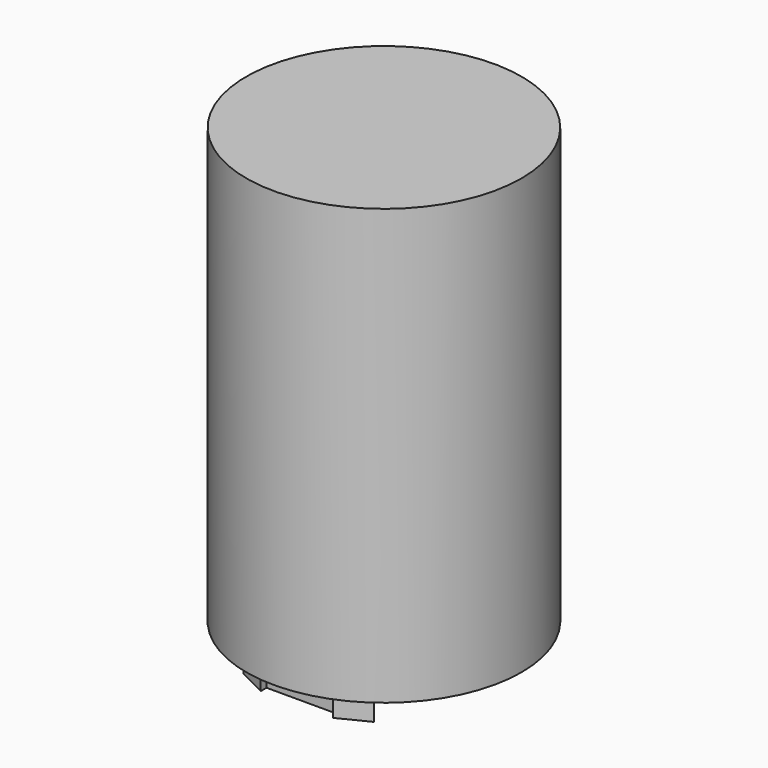
from build123d import *

# Parameters (mm, degrees)
F1_DEPTH = 2
F0_R     = 9.5
F2_DEPTH = 30


with BuildPart() as f1:
    # F0 (on Top) → F1 (new body)
    with BuildSketch(Plane.XY):
        with BuildLine():
            Line((-2.5, -4.5), (-1.5, -4.5))
            Line((-1.5, -4.5), (-1.5, 8))
            ThreePointArc((-1.5, 8), (-1.8805656371, 8.4555551787), (-2.3965696716, 8.1621262073))
            Line((-2.3965696716, 8.1621262073), (-7.1307446703, -4.5))
            Line((-7.1307446703, -4.5), (-6.1307446703, -4.5))
            Line((-6.1307446703, -4.5), (-5.1960329715, -2))
            Line((-5.1960329715, -2), (-2.5, -2))
            Line((-2.5, -2), (-2.5, -4.5))
        make_face()
        Polygon((-2.5, -1), (-4.8221482921, -1), (-2.5, 5.210867734), align=None, mode=Mode.SUBTRACT)
    extrude(amount=-F1_DEPTH)


with BuildPart() as f1b:
    # F0 (on Top) → F1, piece 2 (new body)
    with BuildSketch(Plane.XY):
        with BuildLine():
            Line((1.5, 8.4555551787), (1.5, -4.5))
            ThreePointArc((1.5, -4.5), (5.317050605, -1.9109756291), (7, 2.3832767911))
            ThreePointArc((7, 2.3832767911), (5.154069353, 6.2382818411), (1.5, 8.4555551787))
        make_face()
        Polygon((2.5, -3.0675162561), (2.5, 7.2462004609), (6.0021702136, 2.449122956), align=None, mode=Mode.SUBTRACT)
    extrude(amount=-F1_DEPTH)


with BuildPart() as f1c:
    # F0 (on Top) → F1, piece 3 (new body)
    with BuildSketch(Plane.XY):
        Polygon((2.5, -6), (-2.5, -6), (-2.5, -5.5), (-4.5, -6.5), (-2.5, -7.5), (-2.5, -7), (2.5, -7), (2.5, -7.5), (4.5, -6.5), (2.5, -5.5), align=None)
    extrude(amount=-F1_DEPTH)


with BuildPart() as f2:
    # F0 (on Top) → F2 (new body)
    with BuildSketch(Plane.XY):
        Circle(F0_R)
        Polygon((-2.5, -5.5), (-2.5, -6), (2.5, -6), (2.5, -5.5), (4.5, -6.5), (2.5, -7.5), (2.5, -7), (-2.5, -7), (-2.5, -7.5), (-4.5, -6.5), align=None, mode=Mode.SUBTRACT)
        with BuildLine():
            Line((-1.5, 8), (-1.5, -4.5))
            Line((-1.5, -4.5), (-2.5, -4.5))
            Line((-2.5, -4.5), (-2.5, -2))
            Line((-2.5, -2), (-5.1960329715, -2))
            Line((-5.1960329715, -2), (-6.1307446703, -4.5))
            Line((-6.1307446703, -4.5), (-7.1307446703, -4.5))
            Line((-7.1307446703, -4.5), (-2.3965696716, 8.1621262073))
            ThreePointArc((-2.3965696716, 8.1621262073), (-1.8805656371, 8.4555551787), (-1.5, 8))
        make_face(mode=Mode.SUBTRACT)
        with BuildLine():
            ThreePointArc((7, 2.3832767911), (5.317050605, -1.9109756291), (1.5, -4.5))
            Line((1.5, -4.5), (1.5, 8.4555551787))
            ThreePointArc((1.5, 8.4555551787), (5.154069353, 6.2382818411), (7, 2.3832767911))
        make_face(mode=Mode.SUBTRACT)
        with BuildLine():
            Line((1.5, 8.4555551787), (1.5, -4.5))
            ThreePointArc((1.5, -4.5), (5.317050605, -1.9109756291), (7, 2.3832767911))
            ThreePointArc((7, 2.3832767911), (5.154069353, 6.2382818411), (1.5, 8.4555551787))
        make_face()
        Polygon((2.5, -3.0675162561), (2.5, 7.2462004609), (6.0021702136, 2.449122956), align=None, mode=Mode.SUBTRACT)
        with BuildLine():
            Line((-2.5, -4.5), (-1.5, -4.5))
            Line((-1.5, -4.5), (-1.5, 8))
            ThreePointArc((-1.5, 8), (-1.8805656371, 8.4555551787), (-2.3965696716, 8.1621262073))
            Line((-2.3965696716, 8.1621262073), (-7.1307446703, -4.5))
            Line((-7.1307446703, -4.5), (-6.1307446703, -4.5))
            Line((-6.1307446703, -4.5), (-5.1960329715, -2))
            Line((-5.1960329715, -2), (-2.5, -2))
            Line((-2.5, -2), (-2.5, -4.5))
        make_face()
        Polygon((-2.5, -1), (-4.8221482921, -1), (-2.5, 5.210867734), align=None, mode=Mode.SUBTRACT)
        Polygon((6.0021702136, 2.449122956), (2.5, 7.2462004609), (2.5, -3.0675162561), align=None)
        Polygon((2.5, -6), (-2.5, -6), (-2.5, -5.5), (-4.5, -6.5), (-2.5, -7.5), (-2.5, -7), (2.5, -7), (2.5, -7.5), (4.5, -6.5), (2.5, -5.5), align=None)
        Polygon((-2.5, 5.210867734), (-4.8221482921, -1), (-2.5, -1), align=None)
    extrude(amount=F2_DEPTH)


solid = Compound([f1.part, f1b.part, f1c.part, f2.part])
